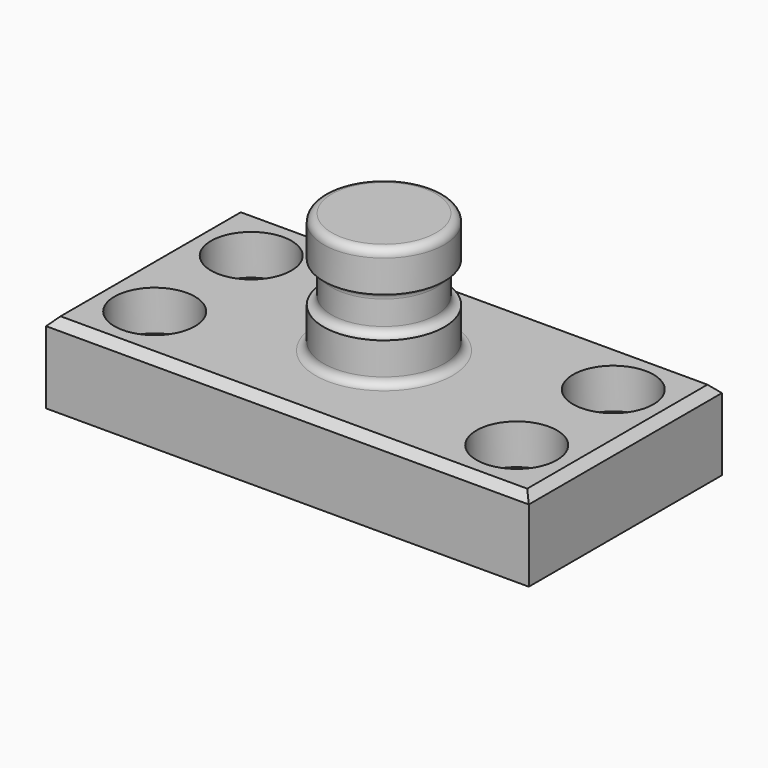
from build123d import *

# Parameters (mm, degrees)
F0_W     = 152.4
F0_H     = 76.2
F1_DEPTH = 25.4
F2_R     = 12.7
F3_DEPTH = 12.7
F4_SIZE  = 2.54
F7_R     = 2.53999


# Not quite as in the source:
# - a fillet or chamfer is up to 0.001 mm smaller than in the source, because OpenCascade refuses the exact size


with BuildPart() as f1:
    # F0 (on Top) → F1 (new body)
    with BuildSketch(Plane.XY):
        Rectangle(F0_W, F0_H)
    extrude(amount=F1_DEPTH)

    # F2 (on face) → F3 (cut)
    with BuildSketch(Plane.XY.offset(25.4)):
        with Locations((57.15, -19.05)):
            Circle(F2_R)
        with Locations((-57.15, -19.05)):
            Circle(F2_R)
        with Locations((-57.15, 19.05)):
            Circle(F2_R)
        with Locations((57.15, 19.05)):
            Circle(F2_R)
    extrude(amount=-F3_DEPTH, mode=Mode.SUBTRACT)

    # F4
    f4_edges = [f1.edges().sort_by_distance(p)[0] for p in [
        (0, -38.1, 25.4),
        (76.2, 0, 25.4),
        (0, 38.1, 25.4),
        (-76.2, 0, 25.4),
    ]]
    chamfer(f4_edges, length=F4_SIZE)

    # F5 (on Front) → F6 (revolve)
    with BuildSketch(Plane.XZ):
        Polygon((0, 63.5), (0, 25.4), (19.05, 25.4), (19.05, 38.1), (16.51, 38.1), (16.51, 50.8), (19.05, 50.8), (19.05, 63.5), align=None)
    revolve(axis=Axis((0, 0, 44.45), (0, 0, 1)))

    # F7 (radius 2.54 in the source; OpenCascade refuses exactly that, so slightly less here)
    f7_edges = [f1.edges().sort_by_distance(p)[0] for p in [
        (-16.51, 0, 38.1),
        (-19.05, 0, 25.4),
        (-16.51, 0, 50.8),
        (-19.05, 0, 63.5),
    ]]
    fillet(f7_edges, radius=F7_R)


solid = f1.part
